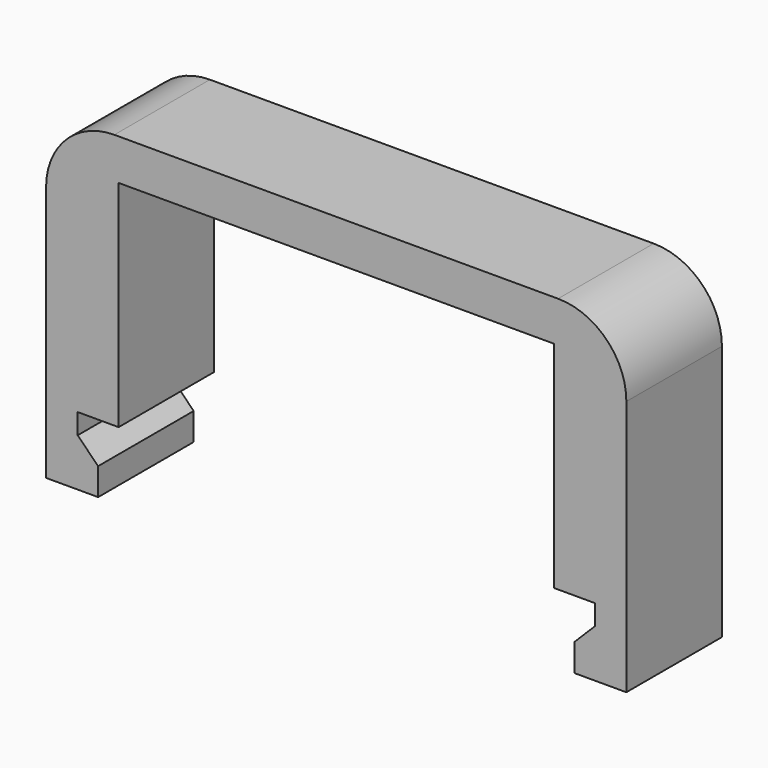
from build123d import *

# Parameters (mm, degrees)
F0_W     = 34
F0_H     = 7
F1_DEPTH = 2.4
F2_W     = 4.25
F2_H     = 16.6
F3_DEPTH = 7
F5_DEPTH = 10
F6_R     = 4


# Not quite as in the source:
# - a pattern or mirror of a feature is missing from the dataset's text; its kind, count and spacing are read off the source's solid


with BuildPart() as f1:
    # F0 (on Top) → F1 (new body)
    with BuildSketch(Plane.XY):
        Rectangle(F0_W, F0_H)
    extrude(amount=F1_DEPTH)

    # F2 (on face) → F3 (join)
    with BuildSketch(Plane(origin=(0, 3.5, 0), x_dir=(-1, 0, 0), z_dir=(0, 1, 0))):
        with Locations((14.875, -8.3)):
            Rectangle(F2_W, F2_H)
        with Locations((-14.875, -8.3)):
            Rectangle(F2_W, F2_H)
    extrude(amount=-F3_DEPTH)

    # F4 (on face) → F5 (cut)
    with BuildSketch(Plane(origin=(0, 3.5, 0), x_dir=(-1, 0, 0), z_dir=(0, 1, 0))):
        Polygon((12.75, -12.6), (12.75, -16.6), (13.95, -16.6), (13.95, -15), (15.15, -13.8), (15.15, -12.6), align=None)
    f5 = extrude(amount=-F5_DEPTH, mode=Mode.SUBTRACT)

    # F5_copies: F5 across plane
    add(f5.mirror(Plane(origin=(0, 0, 0), x_dir=(0, 0, 1), z_dir=(1, 0, 0))), mode=Mode.SUBTRACT)

    # F6
    f6_edges = [f1.edges().sort_by_distance(p)[0] for p in [
        (17, 0, 2.4),
        (-17, 0, 2.4),
    ]]
    fillet(f6_edges, radius=F6_R)


solid = f1.part
